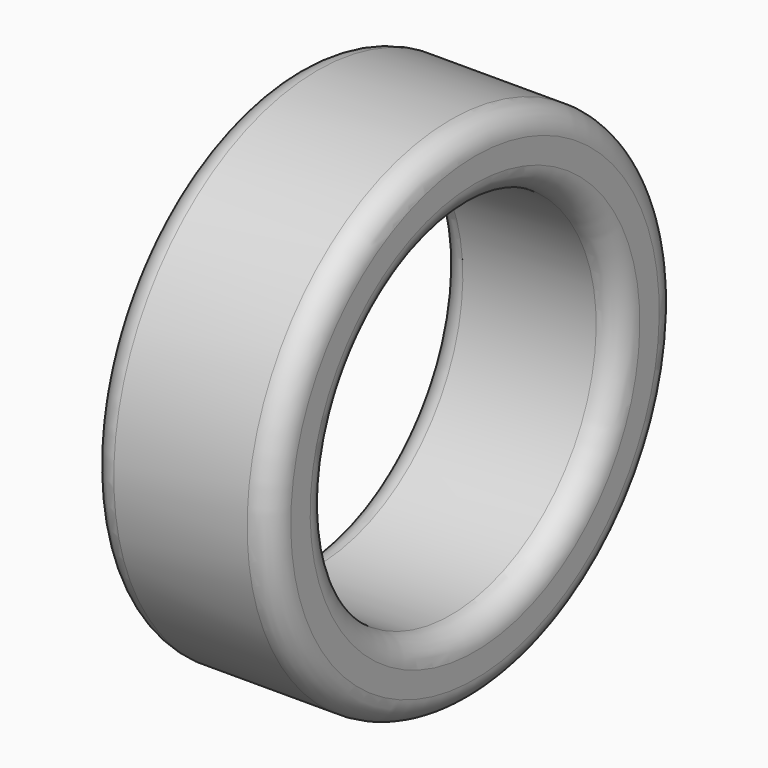
from build123d import *


# Not quite as in the source:
# - the program builds the solid bodies; features that only make, move or delete a surface that nothing else refers to are left out


with BuildPart() as f1:
    # F0 (on Front) → F1 (revolve)
    with BuildSketch(Plane.XZ):
        with BuildLine():
            Line((273.5315602839, 169.9308401752), (-5.8684397161, 169.9308401752))
            ThreePointArc((-5.8684397161, 169.9308401752), (-41.7894642004, 155.0518646595), (-56.6684397161, 119.1308401752))
            Line((-56.6684397161, 119.1308401752), (-56.6684397161, 68.3308401752))
            ThreePointArc((-56.6684397161, 68.3308401752), (-41.7894642004, 32.4098156909), (-5.8684397161, 17.5308401752))
            Line((-5.8684397161, 17.5308401752), (273.5315602839, 17.5308401752))
            ThreePointArc((273.5315602839, 17.5308401752), (309.4525847682, 32.4098156909), (324.3315602839, 68.3308401752))
            Line((324.3315602839, 68.3308401752), (324.3315602839, 119.1308401752))
            ThreePointArc((324.3315602839, 119.1308401752), (309.4525847682, 155.0518646595), (273.5315602839, 169.9308401752))
        make_face()
    revolve(axis=Axis((113.9464541078, 0, -363.4691598248), (1, 0, 0)))


solid = f1.part
